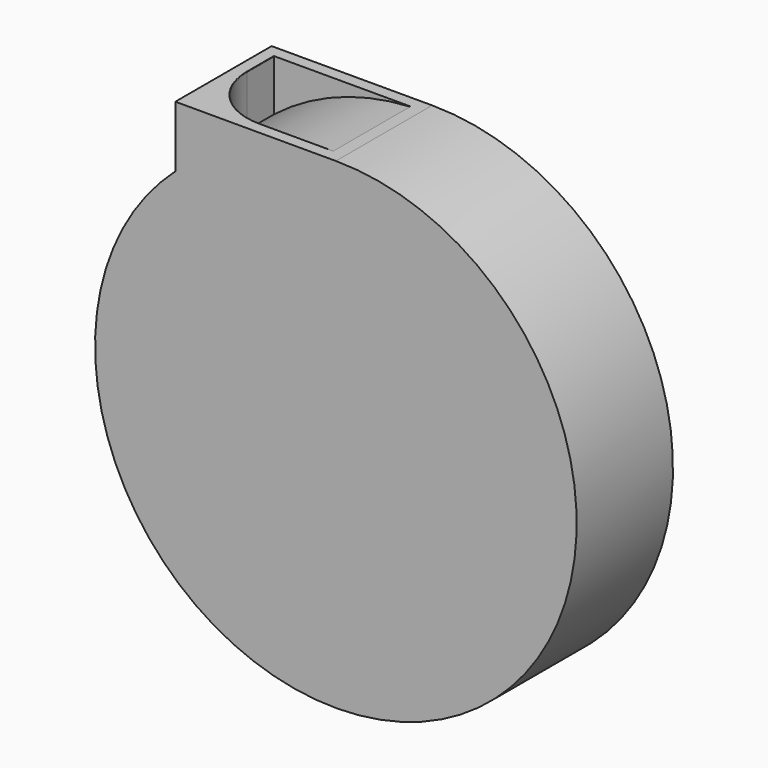
from build123d import *

# Parameters (mm, degrees)
F0_W         = 101.6
F0_H         = 76.2
F1_DEPTH     = 152.4
F2_T         = -7.62
F3_R         = 39.7017420332
F1_FACE_W    = 76.2
F1_FACE_H    = 152.4
F5_T3_ANGLE  = 90
F5_T6_DEPTH  = 21.2582579668
F5_T9_DEPTH  = 46.6582579668
F5_S10_R     = 152.4
F5_T11_DEPTH = 25


# Not quite as in the source:
# - a fillet or chamfer that OpenCascade refuses, or shapes differently, is made with other operations: its cross-section is extruded or revolved along the edge and cut away or added


with BuildPart() as f1:
    # F0 (on Top) → F1 (new body)
    with BuildSketch(Plane.XY):
        with Locations((-6.3440203667, 13.8422726145)):
            Rectangle(F0_W, F0_H)
    extrude(amount=F1_DEPTH)

    # F2
    f2_openings = [f1.faces().sort_by_distance(p)[0] for p in [
        (-6.34402, 13.842273, 152.4),
    ]]
    offset(amount=F2_T, openings=f2_openings)

    # F3
    f3_edges = [f1.edges().sort_by_distance(p)[0] for p in [
        (-49.52402, -16.637727, 80.01),
    ]]
    fillet(f3_edges, radius=F3_R)

    # F1_face (on face) → F4 (revolve)
    with BuildSketch(Plane(origin=(44.4559796333, 13.8422726145, 76.2), x_dir=(0, 1, 0), z_dir=(1, 0, 0))):
        Rectangle(F1_FACE_W, F1_FACE_H)
    revolve(axis=Axis((44.4559796333, 13.8422726145, 0), (0, -1, 0)))

    # F5: fillet of radius 0.2414213562 on 1 edges, made by hand


with BuildPart() as f5_tool1:
    # F5_s2 → F5_t3 (revolve)
    with BuildSketch(Plane.XZ.offset(-23.0640146477)):
        with BuildLine():
            ThreePointArc((-49.7654417229, 152.4), (-49.5947310448, 152.3292893219), (-49.5240203667, 152.1585786438))
            Line((-49.5240203667, 152.1585786438), (-49.5240203667, 152.4))
            Line((-49.5240203667, 152.4), (-49.7654417229, 152.4))
        make_face()
    revolve(axis=Axis((-9.8222783334, 23.0640146477, 152.4), (0, 0, 1)), revolution_arc=F5_T3_ANGLE)


with BuildPart() as f5_tool4:
    # F5_s5 → F5_t6 (new body)
    with BuildSketch(Plane.XZ.offset(-44.3222726145)):
        with BuildLine():
            ThreePointArc((-49.7654417229, 152.4), (-49.5947310448, 152.3292893219), (-49.5240203667, 152.1585786438))
            Line((-49.5240203667, 152.1585786438), (-49.5240203667, 152.4))
            Line((-49.5240203667, 152.4), (-49.7654417229, 152.4))
        make_face()
    extrude(amount=F5_T6_DEPTH)


with BuildPart() as f5_tool7:
    # F5_s8 → F5_t9 (new body)
    with BuildSketch(Plane.YZ.offset(-9.8222783334)):
        with BuildLine():
            ThreePointArc((-16.8791487417, 152.4), (-16.7084380636, 152.3292893219), (-16.6377273855, 152.1585786438))
            Line((-16.6377273855, 152.1585786438), (-16.6377273855, 152.4))
            Line((-16.6377273855, 152.4), (-16.8791487417, 152.4))
        make_face()
    extrude(amount=F5_T9_DEPTH)

    # F5_s10 → F5_t11 (cut, symmetric)
    with BuildSketch(Plane.XZ.offset(16.8)):
        with Locations((44.4559796333, 0)):
            Circle(F5_S10_R)
    extrude(amount=F5_T11_DEPTH, both=True, mode=Mode.SUBTRACT)


with BuildPart() as f1_1:
    add(f1.part)

    # F5_t12: cut F5_tool1, F5_tool4, F5_tool7
    add([f5_tool1.part, f5_tool4.part, f5_tool7.part], mode=Mode.SUBTRACT)


solid = f1_1.part
